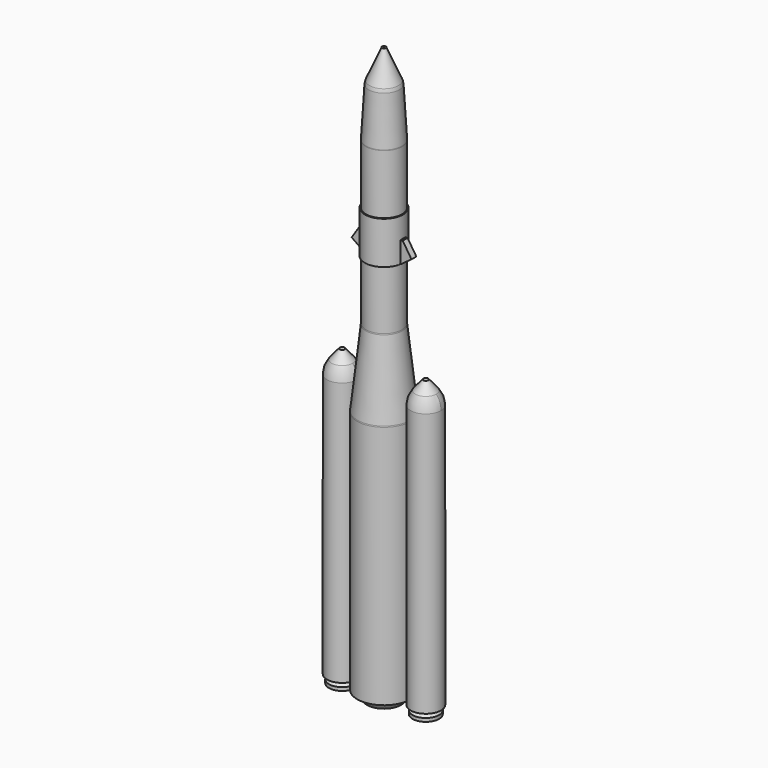
from build123d import *

# Parameters (mm, degrees)
F0_W      = 0.254
F0_H      = 5.3217066717
F0_H_2    = 5.3463475513
F4_R      = 0.5037613029
F5_DEPTH  = 73.7616
F7_R      = 3.81
F8_DEPTH  = 68.072
F12_R     = 5.08
F14_R     = 5.08
F15_DEPTH = 10.4648
F18_R     = 0.1024232424
F21_R     = 0.1039291274
F23_DEPTH = 0.762


# Not quite as in the source:
# - a fillet or chamfer that OpenCascade refuses, or shapes differently, is made with other operations: its cross-section is extruded or revolved along the edge and cut away or added


with BuildPart() as f1:
    # F0 (on Front) → F1 (revolve)
    with BuildSketch(Plane.XZ):
        Polygon((3.81, 66.0637095571), (0, 66.0637095571), (0, -68.1024715304), (5.6330086663, -68.1024715304), (6.6836671904, -68.1024715304), (6.6836671904, -6.5802904429), (4.5427596197, 12.7237095571), (4.5427596197, 27.6973620057), (4.5427596197, 33.0437095571), (4.5427596197, 38.3654162288), (4.5427596197, 53.3637095571), align=None)
        Polygon((5.6330086663, -68.1024715304), (0, -68.1024715304), (0, -71.5639814734), (4.3019275181, -71.5639814734), (4.3019275181, -70.1118931174), align=None)
        with Locations((4.6697596197, 35.7045628929)):
            Rectangle(F0_W, F0_H)
        with Locations((4.6697596197, 30.3705357814)):
            Rectangle(F0_W, F0_H_2)
    revolve(axis=Axis((0, 0, -1.0193809867), (0, 0, -1)))

    # F2 (on Front) → F3 (revolve)
    with BuildSketch(Plane.XZ):
        Polygon((0, 73.6837095571), (0, 66.0637095571), (3.81, 66.0637095571), (0.5037613029, 73.6837095571), align=None)
    revolve(axis=Axis((0, 0, 69.8737095571), (0, 0, 1)))

    # F4 (on Top) → F5 (join)
    with BuildSketch(Plane.XY):
        Circle(F4_R)
        Polygon((-0.2298012114, 0.0951867784), (-0.0951867784, 0.2298012114), (0.0951867784, 0.2298012114), (0.2298012114, 0.0951867784), (0.2298012114, -0.0951867784), (0.0951867784, -0.2298012114), (-0.0951867784, -0.2298012114), (-0.2298012114, -0.0951867784), align=None, mode=Mode.SUBTRACT)
    extrude(amount=F5_DEPTH)

    # F6: fillet of radius 2.54 on 4 edges, made by hand

    # F6_s1 → F6_t2 (revolve)
    with BuildSketch(Plane.XZ):
        with BuildLine():
            ThreePointArc((4.5582378398, 12.5841465207), (4.5466321267, 12.7239236407), (4.5427596197, 12.8641282753))
            Line((4.5427596197, 12.8641282753), (4.4919596197, 12.8641282753))
            Line((4.4919596197, 12.8641282753), (4.4919596197, 12.7209011827))
            Line((4.4919596197, 12.7209011827), (4.5077474042, 12.5785468856))
            Line((4.5077474042, 12.5785468856), (4.5582378398, 12.5841465207))
        make_face()
    revolve(axis=Axis((0, 0, 12.7237095571), (0, 0, -1)))

    # F6_s3 → F6_t4 (revolve, cut)
    with BuildSketch(Plane.XZ):
        with BuildLine():
            ThreePointArc((3.836000085, 65.6130828153), (3.7712853164, 66.0545015234), (3.6303355683, 66.4777882413))
            Line((3.6303355683, 66.4777882413), (3.6769379315, 66.4980085217))
            Line((3.6769379315, 66.4980085217), (3.8601956519, 66.0756482638))
            Line((3.8601956519, 66.0756482638), (3.8867157386, 65.6160089872))
            Line((3.8867157386, 65.6160089872), (3.836000085, 65.6130828153))
        make_face()
    revolve(axis=Axis((0, 0, 66.0637095571), (0, 0, -1)), mode=Mode.SUBTRACT)

    # F6_s5 → F6_t6 (revolve, cut)
    with BuildSketch(Plane.XZ):
        with BuildLine():
            ThreePointArc((4.5427596197, 53.290494478), (4.5417050705, 53.3636791599), (4.5385422987, 53.4368030726))
            Line((4.5385422987, 53.4368030726), (4.5892579522, 53.4397292445))
            Line((4.5892579522, 53.4397292445), (4.5935596197, 53.3651738586))
            Line((4.5935596197, 53.3651738586), (4.5935596197, 53.290494478))
            Line((4.5935596197, 53.290494478), (4.5427596197, 53.290494478))
        make_face()
    revolve(axis=Axis((0, 0, 53.3637095571), (0, 0, -1)), mode=Mode.SUBTRACT)

    # F6_s7 → F6_t8 (revolve, cut)
    with BuildSketch(Plane.XZ):
        with BuildLine():
            ThreePointArc((6.6836671904, -6.7207091612), (6.6797946833, -6.5805045266), (6.6681889703, -6.4407274065))
            Line((6.6681889703, -6.4407274065), (6.7186794058, -6.4351277715))
            Line((6.7186794058, -6.4351277715), (6.7344671904, -6.5774820686))
            Line((6.7344671904, -6.5774820686), (6.7344671904, -6.7207091612))
            Line((6.7344671904, -6.7207091612), (6.6836671904, -6.7207091612))
        make_face()
    revolve(axis=Axis((0, 0, -6.5802904429), (0, 0, -1)), mode=Mode.SUBTRACT)

    # F15 (cut): a face of the model
    f15_faces = [f1.faces().sort_by_distance(p)[0] for p in [
        (0, 0, -71.5639814734),
    ]]
    extrude(f15_faces, amount=-F15_DEPTH, mode=Mode.SUBTRACT)


with BuildPart() as f8:
    # F7 (on Top) → F8 (new body)
    with BuildSketch(Plane.XY):
        with Locations((-10.4936671904, 0)):
            Circle(F7_R)
    extrude(amount=-F8_DEPTH)

    # F10 (on Front) → F11 (revolve)
    with BuildSketch(Plane.XZ):
        Polygon((-11.1376252025, 3.81), (-14.3036671904, 0), (-10.4936671904, 0), (-10.4936671904, 3.81), align=None)
    revolve(axis=Axis((-10.4936671904, 0, 1.905), (0, 0, 1)))

    # F12
    f12_edges = [f8.edges().sort_by_distance(p)[0] for p in [
        (-10.493667, 3.81, 0),
        (-10.493667, -3.81, 0),
    ]]
    fillet(f12_edges, radius=F12_R)

    # F19 (on Front) → F20 (revolve)
    with BuildSketch(Plane.XZ):
        Polygon((-10.4936671904, -68.072), (-12.4853737652, -68.072), (-13.8164749369, -69.2550390959), (-13.8164749369, -70.1118931174), (-10.4936671904, -70.1118931174), align=None)
    revolve(axis=Axis((-10.4936671904, 0, -69.0919465587), (0, 0, -1)))

    # F21
    f21_edges = [f8.edges().sort_by_distance(p)[0] for p in [
        (-7.170859, 0, -69.255039),
    ]]
    fillet(f21_edges, radius=F21_R)


with BuildPart() as f8b:
    # F7 (on Top) → F8, piece 2 (new body)
    with BuildSketch(Plane.XY):
        with BuildLine():
            ThreePointArc((14.3036671904, 0), (10.4936671904, 3.81), (6.6836671904, 0))
            ThreePointArc((6.6836671904, 0), (10.4936671904, -3.81), (14.3036671904, 0))
        make_face()
    extrude(amount=-F8_DEPTH)

    # F9 (on Front) → F13 (revolve)
    with BuildSketch(Plane.XZ):
        Polygon((10.4936671904, 3.81), (10.4936671904, 0), (14.3036671904, 0), (11.1202327535, 3.81), align=None)
    revolve(axis=Axis((10.4936671904, 0, 1.905), (0, 0, 1)))

    # F14
    f14_edges = [f8b.edges().sort_by_distance(p)[0] for p in [
        (6.683667, 0, 0),
    ]]
    fillet(f14_edges, radius=F14_R)

    # F16 (on Front) → F17 (revolve)
    with BuildSketch(Plane.XZ):
        Polygon((12.4905742705, -68.072), (10.4936671904, -68.072), (10.4936671904, -70.1118931174), (13.8262842949, -70.1118931174), (13.8262842949, -69.2455257691), align=None)
    revolve(axis=Axis((10.4936671904, 0, -69.0919465587), (0, 0, -1)))

    # F18
    f18_edges = [f8b.edges().sort_by_distance(p)[0] for p in [
        (7.16105, 0, -69.245526),
    ]]
    fillet(f18_edges, radius=F18_R)


with BuildPart() as f23:
    # F22 (on Front) → F23 (new body, symmetric)
    with BuildSketch(Plane.XZ):
        Polygon((5.2950368583, 33.0758775028), (4.7967596197, 33.0758775028), (4.7967596197, 27.6973620057), (7.5084498966, 29.6675203147), align=None)
    extrude(amount=F23_DEPTH, both=True)


with BuildPart() as f23b:
    # F22 (on Front) → F23, piece 2 (new body, symmetric)
    with BuildSketch(Plane.XZ):
        Polygon((-7.4954263578, 29.6580581599), (-4.7967596197, 27.6973620057), (-4.7967596197, 33.0313891172), (-5.3047596197, 33.0313891172), align=None)
    extrude(amount=F23_DEPTH, both=True)


solid = Compound([f1.part, f8.part, f8b.part, f23.part, f23b.part])
